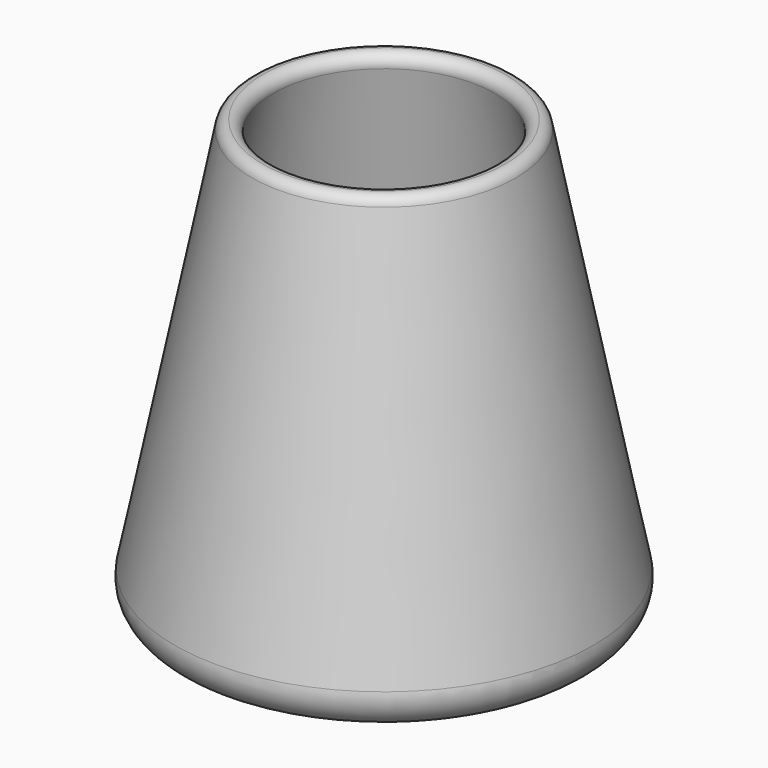
from build123d import *

# Parameters (mm, degrees)
F0_R = 50
F2_R = 30
F4_T = -5
F5_R = 2.49999
F6_R = 7.5


# Not quite as in the source:
# - a fillet or chamfer is up to 0.001 mm smaller than in the source, because OpenCascade refuses the exact size


with BuildPart() as f3:
    # F0 (on Top) → F3 section 0
    with BuildSketch(Plane.XY):
        Circle(F0_R)
    # F2 (on offset) → F3 section 1
    with BuildSketch(Plane.XY.offset(100)):
        Circle(F2_R)
    loft()

    # F4
    f4_openings = [f3.faces().sort_by_distance(p)[0] for p in [
        (0, 0, 100),
    ]]
    offset(amount=F4_T, openings=f4_openings, kind=Kind.INTERSECTION)

    # F5 (radius 2.5 in the source; OpenCascade refuses exactly that, so slightly less here)
    f5_edges = [f3.edges().sort_by_distance(p)[0] for p in [
        (-30, 0, 100),
        (-24.90098, 0, 100),
    ]]
    fillet(f5_edges, radius=F5_R)

    # F6
    f6_edges = [f3.edges().sort_by_distance(p)[0] for p in [
        (-50, 0, 0),
        (-43.90098, 0, 5),
    ]]
    fillet(f6_edges, radius=F6_R)


solid = f3.part
